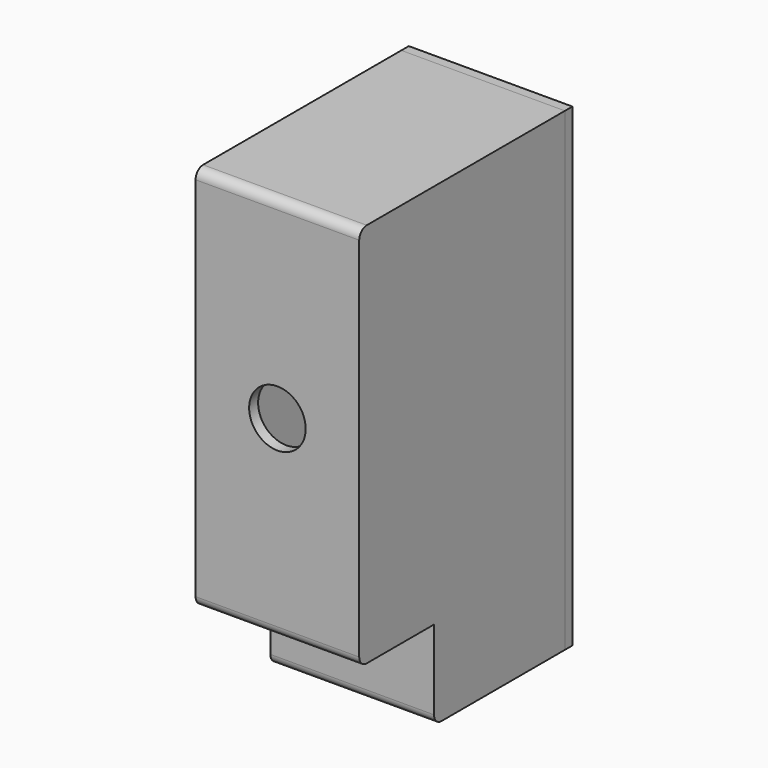
from build123d import *

# Parameters (mm, degrees)
F1_DEPTH  = 35
F2_R      = 2
F3_T      = -2.4
F4_R      = 6.05
F5_DEPTH  = 55.001
F6_W      = 29.5
F6_H      = 96
F7_DEPTH  = 1.5
F6_W_2    = 35
F6_H_2    = 101.5
F6_W_3    = 30.2
F6_H_3    = 96.7
F8_DEPTH  = 2
F9_R      = 1.75
F10_DEPTH = 51.1
F11_START = 17.6
F11_DEPTH = 33.5
F12_R     = 2.35
F13_DEPTH = 57.001
F14_R     = 2.15
F15_DEPTH = 57.001


with BuildPart() as f1:
    # F0 (on Right) → F1 (new body)
    with BuildSketch(Plane.YZ):
        Polygon((20, 19), (20, 0), (55, 0), (55, 101.5), (0, 101.5), (0, 19), align=None)
    extrude(amount=F1_DEPTH)

    # F2
    f2_edges = [f1.edges().sort_by_distance(p)[0] for p in [
        (17.5, 0, 101.5),
        (17.5, 0, 19),
        (17.5, 20, 0),
    ]]
    fillet(f2_edges, radius=F2_R)

    # F3
    f3_openings = [f1.faces().sort_by_distance(p)[0] for p in [
        (17.5, 55, 50.75),
    ]]
    offset(amount=F3_T, openings=f3_openings, kind=Kind.INTERSECTION)

    # F4 (on face) → F5 (cut, through all)
    with BuildSketch(Plane.XZ):
        with Locations((17.5, 60.25)):
            Circle(F4_R)
    extrude(amount=-F5_DEPTH, mode=Mode.SUBTRACT)

    # F9 (on face) → F10 (join, through all)
    with BuildSketch(Plane(origin=(0, 2.4, 0), x_dir=(-1, 0, 0), z_dir=(0, 1, 0))):
        with BuildLine():
            Line((-2.4, 99.1), (-10.4, 99.1))
            ThreePointArc((-10.4, 99.1), (-8.0568542495, 93.4431457505), (-2.4, 91.1))
            Line((-2.4, 91.1), (-2.4, 99.1))
        make_face()
        with Locations((-5.2284271247, 96.2715728753)):
            Circle(F9_R, mode=Mode.SUBTRACT)
        with BuildLine():
            Line((-24.6, 99.1), (-32.6, 99.1))
            Line((-32.6, 99.1), (-32.6, 91.1))
            ThreePointArc((-32.6, 91.1), (-26.9431457505, 93.4431457505), (-24.6, 99.1))
        make_face()
        with Locations((-29.7715728753, 96.2715728753)):
            Circle(F9_R, mode=Mode.SUBTRACT)
    extrude(amount=F10_DEPTH)

    # F9 (on face) → F11 (join)
    with BuildSketch(Plane(origin=(0, 2.4, 0), x_dir=(-1, 0, 0), z_dir=(0, 1, 0)).offset(F11_START)):
        with BuildLine():
            ThreePointArc((-24.6, 2.4), (-26.9431457505, 8.0568542495), (-32.6, 10.4))
            Line((-32.6, 10.4), (-32.6, 2.4))
            Line((-32.6, 2.4), (-24.6, 2.4))
        make_face()
        with Locations((-29.7715728753, 5.2284271247)):
            Circle(F9_R, mode=Mode.SUBTRACT)
        with BuildLine():
            Line((-2.4, 2.4), (-2.4, 10.4))
            ThreePointArc((-2.4, 10.4), (-8.0568542495, 8.0568542495), (-10.4, 2.4))
            Line((-10.4, 2.4), (-2.4, 2.4))
        make_face()
        with Locations((-5.2284271247, 5.2284271247)):
            Circle(F9_R, mode=Mode.SUBTRACT)
    extrude(amount=F11_DEPTH)


with BuildPart() as f7:
    # F6 (on face) → F7 (new body)
    with BuildSketch(Plane(origin=(0, 55, 0), x_dir=(-1, 0, 0), z_dir=(0, 1, 0))):
        with Locations((-17.5, 50.75)):
            Rectangle(F6_W, F6_H)
    extrude(amount=-F7_DEPTH)

    # F6 (on face) → F8 (join)
    with BuildSketch(Plane(origin=(0, 55, 0), x_dir=(-1, 0, 0), z_dir=(0, 1, 0))):
        with Locations((-17.5, 50.75)):
            Rectangle(F6_W_2, F6_H_2)
        with Locations((-17.5, 50.75)):
            Rectangle(F6_W_3, F6_H_3, mode=Mode.SUBTRACT)
        with Locations((-17.5, 50.75)):
            Rectangle(F6_W_3, F6_H_3)
        with Locations((-17.5, 50.75)):
            Rectangle(F6_W, F6_H, mode=Mode.SUBTRACT)
        with Locations((-17.5, 50.75)):
            Rectangle(F6_W, F6_H)
    extrude(amount=F8_DEPTH)

    # F12 (on face) → F13 (cut, through all)
    with BuildSketch(Plane(origin=(0, 57, 0), x_dir=(-1, 0, 0), z_dir=(0, 1, 0))):
        with Locations((-5.2284271247, 96.2715728753)):
            Circle(F12_R)
        with Locations((-29.7715728753, 96.2715728753)):
            Circle(F12_R)
        with Locations((-29.7715728753, 5.2284271247)):
            Circle(F12_R)
        with Locations((-5.2284271247, 5.2284271247)):
            Circle(F12_R)
    extrude(amount=-F13_DEPTH, mode=Mode.SUBTRACT)

    # F14 (on face) → F15 (cut, through all)
    with BuildSketch(Plane(origin=(0, 57, 0), x_dir=(-1, 0, 0), z_dir=(0, 1, 0))):
        with Locations((-25.5, 86.5)):
            Circle(F14_R)
        with Locations((-9.5, 86.5)):
            Circle(F14_R)
        with Locations((-25.5, 62.6666666667)):
            Circle(F14_R)
        with Locations((-9.5, 62.6666666667)):
            Circle(F14_R)
        with Locations((-25.5, 38.8333333333)):
            Circle(F14_R)
        with Locations((-9.5, 38.8333333333)):
            Circle(F14_R)
        with Locations((-25.5, 15)):
            Circle(F14_R)
        with Locations((-9.5, 15)):
            Circle(F14_R)
    extrude(amount=-F15_DEPTH, mode=Mode.SUBTRACT)


solid = Compound([f1.part, f7.part])
